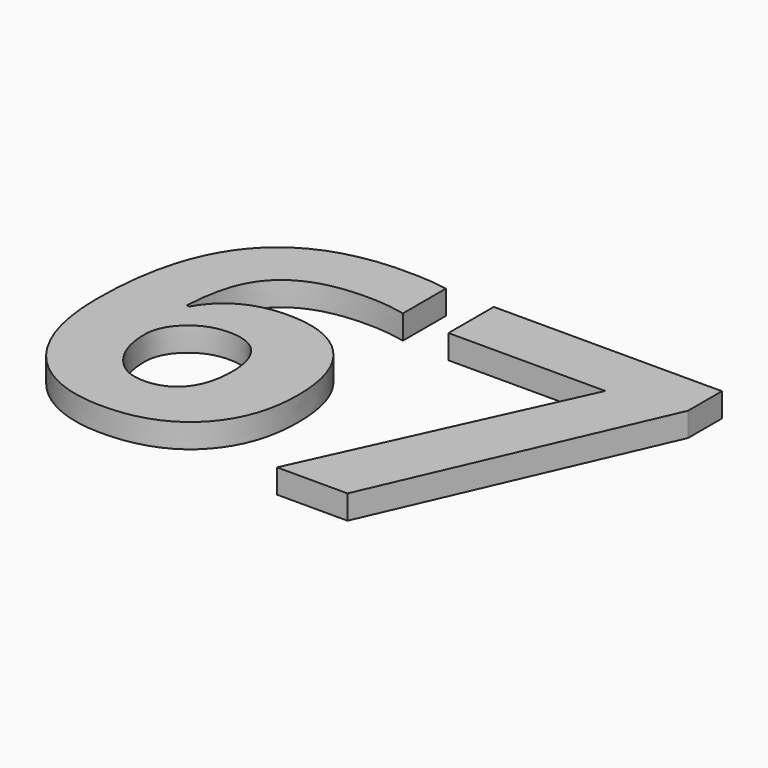
from build123d import *

# Parameters (mm, degrees)
F0_TEXT_SIZE = 111.1111111111
F1_DEPTH     = 6


# Not quite as in the source:
# - Text() gives the source's letters only with a copy of the font that has no kerning and outlines rounded to 1/6400 em; it was checked with that copy


with BuildPart() as f1:
    # F0 (on Top) → F1 (new body)
    with BuildSketch(Plane.XY):
        with Locations((-52.7461134336, -59.9999996942)):
            Text('67', F0_TEXT_SIZE, font='Open Sans', font_style=FontStyle.BOLD, text_align=(TextAlign.LEFT, TextAlign.BOTTOM))
    extrude(amount=F1_DEPTH)


solid = f1.part
